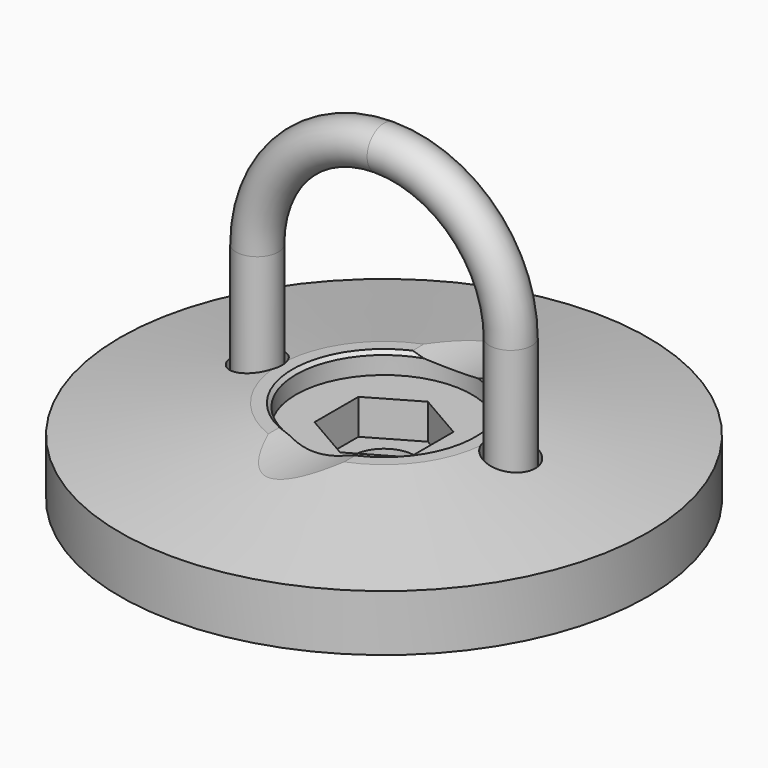
from build123d import *

# Parameters (mm, degrees)
F2_SIZE         = 0.5
F3_R            = 15
F4_DEPTH        = 50
F8_R            = 3
F12_D           = 7
F12_DEPTH       = 5.5
F12_TIP         = 2.1030121666
F14_D           = 4.5
F14_CBORE_D     = 9
F14_CBORE_DEPTH = 5
F15_D           = 8.8
F15_CSINK_D     = 9.5
F15_CSINK_ANGLE = 90
F17_DEPTH       = 5


# Not quite as in the source:
# - a feature of the source that left no trace in its solid (it failed there, or was rolled back) is left out


with BuildPart() as f1:
    # F0 (on Front) → F1 (revolve)
    with BuildSketch(Plane.XZ):
        Polygon((-37.5, 0), (0, 0), (0, 9), (-12.5, 9), (-12.5, 12), (-14.8148727215, 12), (-37.5, 8), align=None)
    revolve(axis=Axis((0, 0, 21.8192628079), (0, 0, 1)))

    # F2
    f2_edges = [f1.edges().sort_by_distance(p)[0] for p in [
        (12.5, 0, 12),
    ]]
    chamfer(f2_edges, length=F2_SIZE)


with BuildPart() as f4:
    # F3 (on Front) → F4 (new body, symmetric)
    with BuildSketch(Plane.XZ):
        with Locations((0, 26)):
            Circle(F3_R)
    extrude(amount=F4_DEPTH, both=True)


with BuildPart() as f1_1:
    add(f1.part)

    # F5: cut F4
    add(f4.part, mode=Mode.SUBTRACT)

    # F12 (one way)
    with BuildSketch(Plane(origin=(0, 0, 8), x_dir=(1, 0, 0), z_dir=(0, 0, -1))):
        with Locations((-18, 0), (18, 0)):
            Circle(F12_D / 2)
    extrude(amount=-F12_DEPTH, mode=Mode.SUBTRACT)
    with Locations(Plane(origin=(0, 0, 8), x_dir=(1, 0, 0), z_dir=(0, 0, -1))):
        with Locations((-18, 0), (18, 0)):
            with Locations((0, 0, -(F12_DEPTH + F12_TIP / 2))):  # 118° drill point
                Cone(0, F12_D / 2, F12_TIP, mode=Mode.SUBTRACT)

    # F14 (through all)
    with Locations(Plane(origin=(0, 0, 0), x_dir=(1, 0, 0), z_dir=(0, 0, -1))):
        with Locations((-18, 0), (18, 0)):
            CounterBoreHole(F14_D / 2, F14_CBORE_D / 2, F14_CBORE_DEPTH)

    # F15 (through all)
    with Locations(Plane(origin=(0, 0, 0), x_dir=(1, 0, 0), z_dir=(0, 0, -1))):
        with Locations((0, 0)):
            CounterSinkHole(F15_D / 2, F15_CSINK_D / 2, counter_sink_angle=F15_CSINK_ANGLE)

    # F16 (on face) → F17 (cut)
    with BuildSketch(Plane.XY.offset(9)):
        Polygon((6.75, 3.897114317), (0, 7.7942286341), (-6.75, 3.897114317), (-6.75, -3.897114317), (0, -7.7942286341), (6.75, -3.897114317), align=None)
    extrude(amount=-F17_DEPTH, mode=Mode.SUBTRACT)


with BuildPart() as f9:
    # F9: sweep along a path in F6
    with BuildLine(Plane.XZ) as f9_path:
        Line((-18, 9), (-18, 26))
        ThreePointArc((-18, 26), (-12.7279220614, 38.7279220614), (0, 44))
        ThreePointArc((0, 44), (12.7279220614, 38.7279220614), (18, 26))
        Line((18, 26), (18, 9))
    # F8 (on line) → F9 (sweep)
    with BuildSketch(Plane(origin=(0, 0, 9), x_dir=(1, 0, 0), z_dir=(0, 0, -1))):
        with Locations((-18, 0)):
            Circle(F8_R)
    sweep(path=f9_path.line)


solid = Compound([f1_1.part, f9.part])
